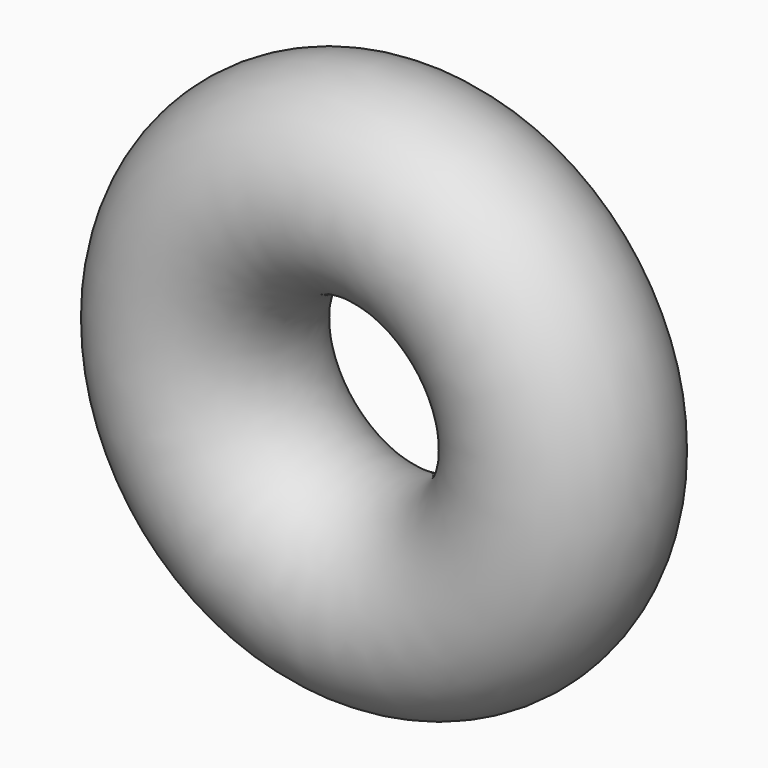
from build123d import *

# Parameters (mm, degrees)
F0_R = 11.1797222355


# Not quite as in the source:
# - the program builds the solid bodies; features that only make, move or delete a surface that nothing else refers to are left out


with BuildPart() as f2:
    # F0 (on Top) → F2 (revolve)
    with BuildSketch(Plane.XY):
        with Locations((-62.280677259, 52.5233596563)):
            Circle(F0_R)
    revolve(axis=Axis((-82.9103291035, 50.9820729494, 0), (0, -1, 0)))


solid = f2.part
